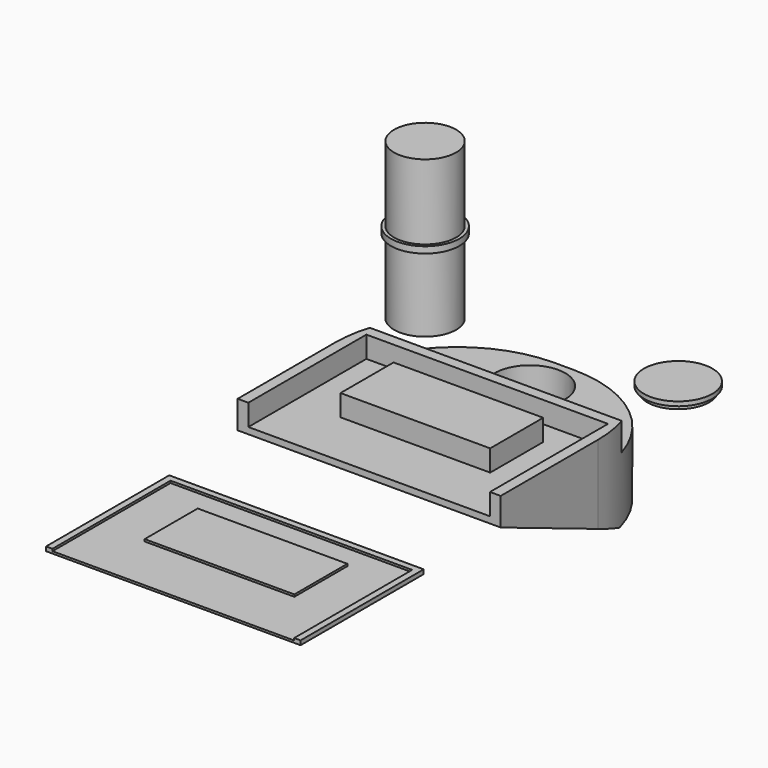
from build123d import *

# Parameters (mm, degrees)
F0_R      = 14.5
F1_DEPTH  = 35
F2_R      = 16
F3_DEPTH  = 3
F4_R      = 14.5
F5_DEPTH  = 35
F6_W      = 113
F6_H      = 69
F7_DEPTH  = 3
F8_W      = 70
F8_H      = 31
F9_DEPTH  = 10
F10_W     = 69
F10_H     = 13
F11_DEPTH = 5
F12_W     = 118
F12_H     = 13
F13_DEPTH = 5
F14_W     = 74
F14_H     = 13
F15_DEPTH = 5
F16_W     = 123
F16_H     = 74
F17_DEPTH = 30
F18_W     = 123
F18_H     = 30
F19_DEPTH = 40
F20_R     = 16.5
F21_DEPTH = 30.001
F22_SIZE2 = 72
F22_SIZE  = 30
F23_R     = 57
F24_R     = 57
F25_R     = 3
F26_DEPTH = 114.001
F27_R     = 14.5
F28_DEPTH = 2
F29_R     = 16
F30_DEPTH = 2
F31_W     = 119
F31_H     = 72
F32_DEPTH = 1
F33_W     = 3
F33_H     = 3
F33_W_2   = 113
F33_H_2   = 69
F34_DEPTH = 1
F35_W     = 70
F35_H     = 31
F36_DEPTH = 1


with BuildPart() as f1:
    # F0 (on Top) → F1 (new body)
    with BuildSketch(Plane.XY):
        with Locations((-51.4401979744, 51.072768867)):
            Circle(F0_R)
    extrude(amount=F1_DEPTH)

    # F2 (on face) → F3 (join)
    with BuildSketch(Plane.XY.offset(35)):
        with Locations((-51.4401979744, 51.072768867)):
            Circle(F2_R)
    extrude(amount=F3_DEPTH)

    # F4 (on face) → F5 (join)
    with BuildSketch(Plane.XY.offset(38)):
        with Locations((-51.4401979744, 51.072768867)):
            Circle(F4_R)
    extrude(amount=F5_DEPTH)


with BuildPart() as f7:
    # F6 (on Top) → F7 (new body)
    with BuildSketch(Plane.XY):
        with Locations((11.9167239517, -26.3256993649)):
            Rectangle(F6_W, F6_H)
    extrude(amount=F7_DEPTH)

    # F8 (on face) → F9 (join)
    with BuildSketch(Plane.XY.offset(3)):
        with Locations((11.9167239517, -18.3256993649)):
            Rectangle(F8_W, F8_H)
    extrude(amount=F9_DEPTH)

    # F10 (on face) → F11 (join)
    with BuildSketch(Plane.YZ.offset(68.4167239517)):
        with Locations((-26.3256993649, 6.5)):
            Rectangle(F10_W, F10_H)
    extrude(amount=F11_DEPTH)

    # F12 (on face) → F13 (join)
    with BuildSketch(Plane(origin=(0, 8.1743006351, 0), x_dir=(-1, 0, 0), z_dir=(0, 1, 0))):
        with Locations((-14.4167239517, 6.5)):
            Rectangle(F12_W, F12_H)
    extrude(amount=F13_DEPTH)

    # F14 (on face) → F15 (join)
    with BuildSketch(Plane(origin=(-44.5832760483, 0, 0), x_dir=(0, -1, 0), z_dir=(-1, 0, 0))):
        with Locations((23.8256993649, 6.5)):
            Rectangle(F14_W, F14_H)
    extrude(amount=F15_DEPTH)

    # F16 (on face) → F17 (join)
    with BuildSketch(Plane(origin=(0, 0, 0), x_dir=(1, 0, 0), z_dir=(0, 0, -1))):
        with Locations((11.9167239517, 23.8256993649)):
            Rectangle(F16_W, F16_H)
    extrude(amount=F17_DEPTH)

    # F18 (on face) → F19 (join)
    with BuildSketch(Plane(origin=(0, 13.1743006351, 0), x_dir=(-1, 0, 0), z_dir=(0, 1, 0))):
        with Locations((-11.9167239517, -15)):
            Rectangle(F18_W, F18_H)
    extrude(amount=F19_DEPTH)

    # F20 (on face) → F21 (cut, through all)
    with BuildSketch(Plane.XY):
        with Locations((11.9167239517, 33.1743006351)):
            Circle(F20_R)
    extrude(amount=-F21_DEPTH, mode=Mode.SUBTRACT)

    # F22
    f22_edges = [f7.edges().sort_by_distance(p)[0] for p in [
        (11.916724, -60.825699, -30),
    ]]
    chamfer(f22_edges, length=F22_SIZE, length2=F22_SIZE2)

    # F23
    f23_edges = [f7.edges().sort_by_distance(p)[0] for p in [
        (73.416724, 53.174301, -15),
    ]]
    fillet(f23_edges, radius=F23_R)

    # F24
    f24_edges = [f7.edges().sort_by_distance(p)[0] for p in [
        (-49.583276, 53.174301, -15),
    ]]
    fillet(f24_edges, radius=F24_R)

    # F25 (on face) → F26 (cut, through all)
    with BuildSketch(Plane(origin=(0, 53.1743006351, 0), x_dir=(-1, 0, 0), z_dir=(0, 1, 0))):
        with Locations((-11.9167239517, -15)):
            Circle(F25_R)
    extrude(amount=-F26_DEPTH, mode=Mode.SUBTRACT)


with BuildPart() as f28:
    # F27 (on Top) → F28 (new body)
    with BuildSketch(Plane.XY):
        with Locations((56.549821049, 64.0196353197)):
            Circle(F27_R)
    extrude(amount=F28_DEPTH)

    # F29 (on face) → F30 (join)
    with BuildSketch(Plane.XY.offset(2)):
        with Locations((56.549821049, 64.0196353197)):
            Circle(F29_R)
    extrude(amount=F30_DEPTH)


with BuildPart() as f32:
    # F31 (on Top) → F32 (new body)
    with BuildSketch(Plane.XY):
        with Locations((15.024092472, -143.1891386509)):
            Rectangle(F31_W, F31_H)
    extrude(amount=F32_DEPTH)

    # F33 (on face) → F34 (join)
    with BuildSketch(Plane.XY.offset(1)):
        with Locations((-42.975907528, -108.6891386509)):
            Rectangle(F33_W, F33_H)
        with Locations((15.024092472, -108.6891386509)):
            Rectangle(F33_W_2, F33_H)
        with Locations((-42.975907528, -144.6891386509)):
            Rectangle(F33_W, F33_H_2)
        with Locations((73.024092472, -108.6891386509)):
            Rectangle(F33_W, F33_H)
        with Locations((73.024092472, -144.6891386509)):
            Rectangle(F33_W, F33_H_2)
    extrude(amount=F34_DEPTH)

    # F35 (on face) → F36 (join)
    with BuildSketch(Plane.XY.offset(1)):
        with Locations((15.024092472, -136.6891386509)):
            Rectangle(F35_W, F35_H)
    extrude(amount=F36_DEPTH)


solid = Compound([f1.part, f7.part, f28.part, f32.part])
